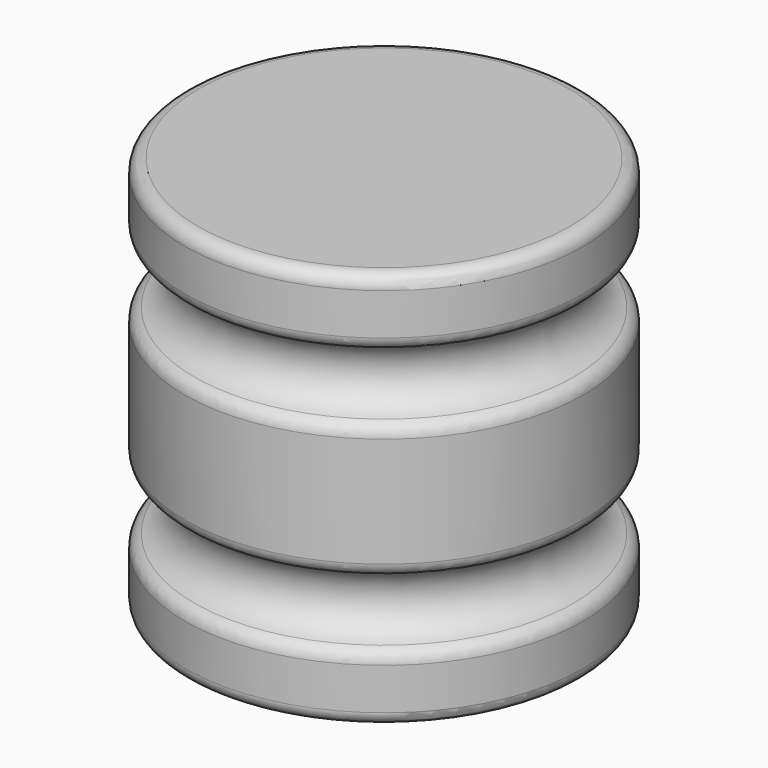
from build123d import *

# Parameters (mm, degrees)
F2_R = 2.54


with BuildPart() as f1:
    # F0 (on Front) → F1 (revolve)
    with BuildSketch(Plane.XZ):
        with BuildLine():
            Line((-38.1, 0), (0, 0))
            Line((0, 0), (0, 12.7))
            ThreePointArc((0, 12.7), (-6.35, 19.05), (0, 25.4))
            Line((0, 25.4), (0, 50.8))
            ThreePointArc((0, 50.8), (-6.35, 57.15), (0, 63.5))
            Line((0, 63.5), (0, 76.2))
            Line((0, 76.2), (-38.1, 76.2))
            Line((-38.1, 76.2), (-38.1, 0))
        make_face()
    revolve(axis=Axis((-38.1, 0, 38.1), (0, 0, 1)))

    # F2
    f2_edges = [f1.edges().sort_by_distance(p)[0] for p in [
        (-76.2, 0, 76.2),
        (-76.2, 0, 63.5),
        (-76.2, 0, 25.4),
        (-76.2, 0, 0),
        (-76.2, 0, 12.7),
        (-76.2, 0, 50.8),
    ]]
    fillet(f2_edges, radius=F2_R)


solid = f1.part
